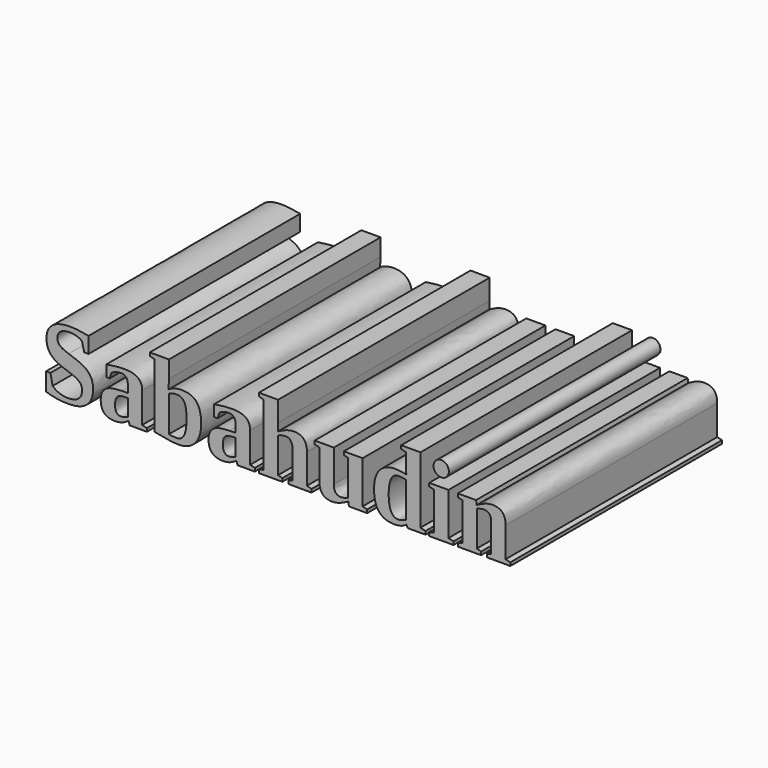
from build123d import *

# Parameters (mm, degrees)
F1_TEXT_SIZE = 19.3055369352
F2_DEPTH     = 50


# Not quite as in the source:
# - Text() gives the source's letters only with a copy of the font that has no kerning and outlines rounded to 1/6400 em; it was checked with that copy


with BuildPart() as f2:
    # F1 (on face) → F2 (new body)
    with BuildSketch(Plane.XZ):
        with Locations((-66.3066615755, 42.5814562254)):
            Text('Sabahudin', F1_TEXT_SIZE, font='Tinos', font_style=FontStyle.BOLD, text_align=(TextAlign.LEFT, TextAlign.BOTTOM))
    extrude(amount=F2_DEPTH)


solid = f2.part
